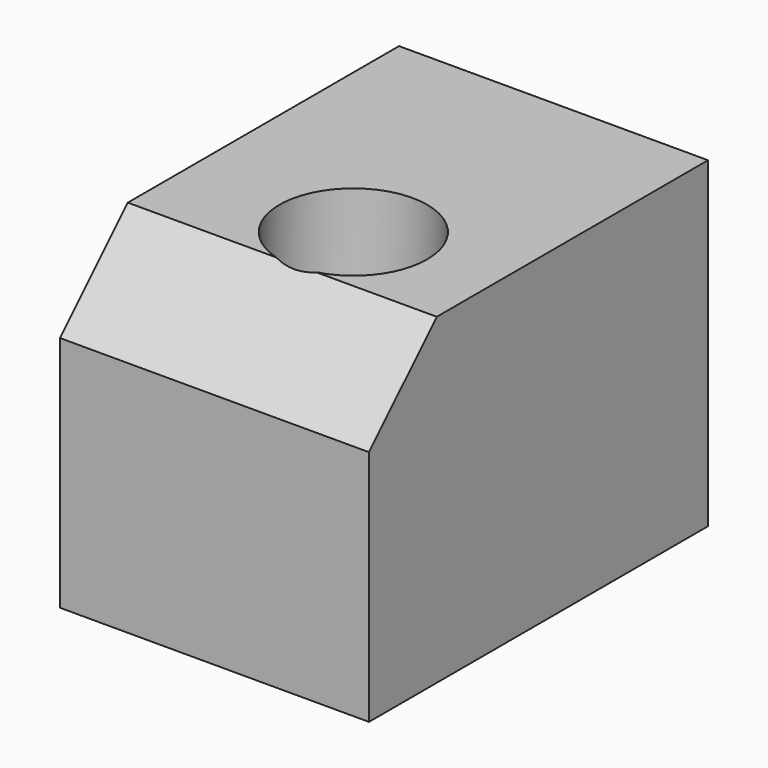
from build123d import *

# Parameters (mm, degrees)
F0_W        = 92.6014147699
F0_H        = 96.5672135353
F1_DEPTH    = 127
F2_R        = 22.1483335528
F3_DEPTH    = 25.4
F4_T1_DEPTH = 223.2429105586


# Not quite as in the source:
# - a fillet or chamfer that OpenCascade refuses, or shapes differently, is made with other operations: its cross-section is extruded or revolved along the edge and cut away or added


with BuildPart() as f1:
    # F0 (on Front) → F1 (new body)
    with BuildSketch(Plane.XZ):
        with Locations((0.2974327654, -0.594869256)):
            Rectangle(F0_W, F0_H)
    extrude(amount=F1_DEPTH)

    # F2 (on face) → F3 (cut)
    with BuildSketch(Plane.XY.offset(47.6887375116)):
        with Locations((4.5238654129, -80.271743238)):
            Circle(F2_R)
    extrude(amount=-F3_DEPTH, mode=Mode.SUBTRACT)

    # F4: chamfer of 25.4 on 1 edges, made by hand

    # F4_s2 → F4_t1 (cut)
    with BuildSketch(Plane.YZ.offset(-111.3240225139)):
        Polygon((-101.6, 47.6887375116), (-127, 22.2887375116), (-127, 47.6887375116), align=None)
    extrude(amount=F4_T1_DEPTH, mode=Mode.SUBTRACT)


solid = f1.part
